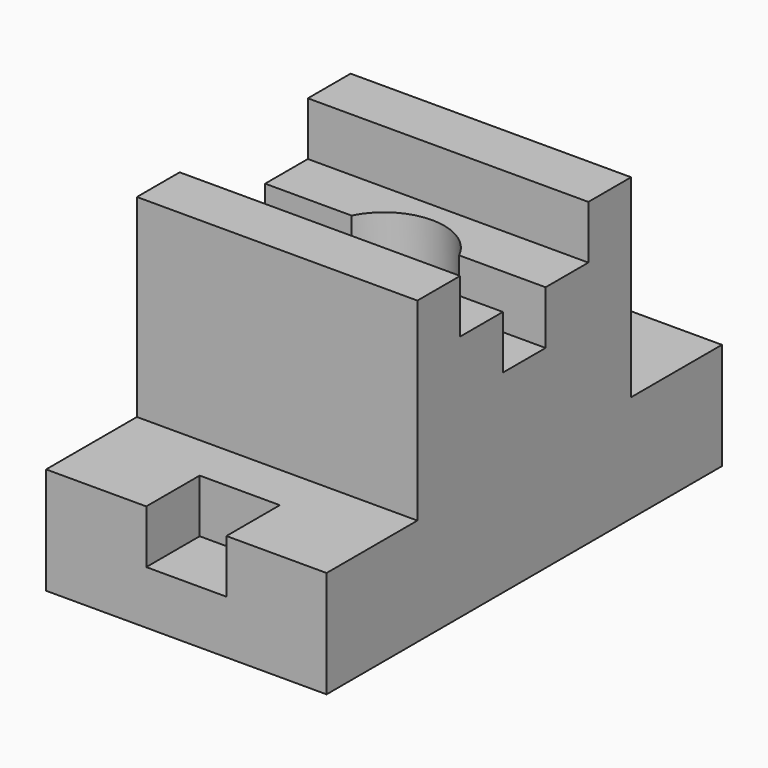
from build123d import *

# Parameters (mm, degrees)
F1_DEPTH = 21
F2_R     = 9
F3_DEPTH = 8
F4_W     = 12
F4_H     = 10
F5_DEPTH = 8


# Not quite as in the source:
# - a pattern or mirror of a feature is missing from the dataset's text; its kind, count and spacing are read off the source's solid


with BuildPart() as f1:
    # F0 (on Right) → F1 (new body, symmetric)
    with BuildSketch(Plane.YZ):
        Polygon((-37, 0), (0, 0), (37, 0), (37, 16), (20, 16), (20, 45), (12, 45), (12, 37), (4, 37), (4, 29), (0, 29), (-4, 29), (-4, 37), (-12, 37), (-12, 45), (-20, 45), (-20, 16), (-37, 16), align=None)
    extrude(amount=F1_DEPTH, both=True)

    # F2 (on face) → F3 (cut, through all)
    with BuildSketch(Plane.XY.offset(37)):
        Circle(F2_R)
    extrude(amount=-F3_DEPTH, mode=Mode.SUBTRACT)

    # F4 (on face) → F5 (cut)
    with BuildSketch(Plane.XY.offset(16)):
        with Locations((0, -32)):
            Rectangle(F4_W, F4_H)
    f5 = extrude(amount=-F5_DEPTH, mode=Mode.SUBTRACT)

    # F5_copies: F5 across plane
    add(f5.mirror(Plane.ZX), mode=Mode.SUBTRACT)


solid = f1.part
